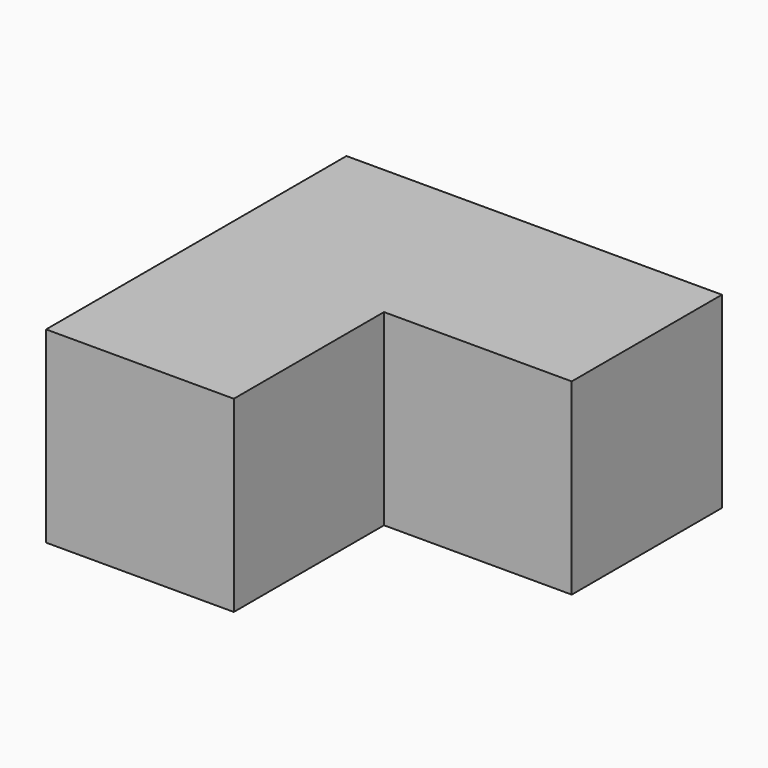
from build123d import *

# Parameters (mm, degrees)
F1_W     = 101.6
F1_H     = 101.6
F2_DEPTH = 101.6
F3_W     = 101.6
F3_H     = 101.6
F4_DEPTH = 101.6


# Not quite as in the source:
# - a variable given as a bare number and used for a length is read in inches; the dataset says mm whatever the document's units were


with BuildPart() as f2:
    # F1 (on Front) → F2 (new body, symmetric)
    with BuildSketch(Plane.XZ):
        Rectangle(F1_W, F1_H)
    extrude(amount=F2_DEPTH, both=True)

    # F3 (on face) → F4 (join)
    with BuildSketch(Plane.YZ.offset(50.8)):
        with Locations((50.8, 0)):
            Rectangle(F3_W, F3_H)
    extrude(amount=F4_DEPTH)


solid = f2.part
